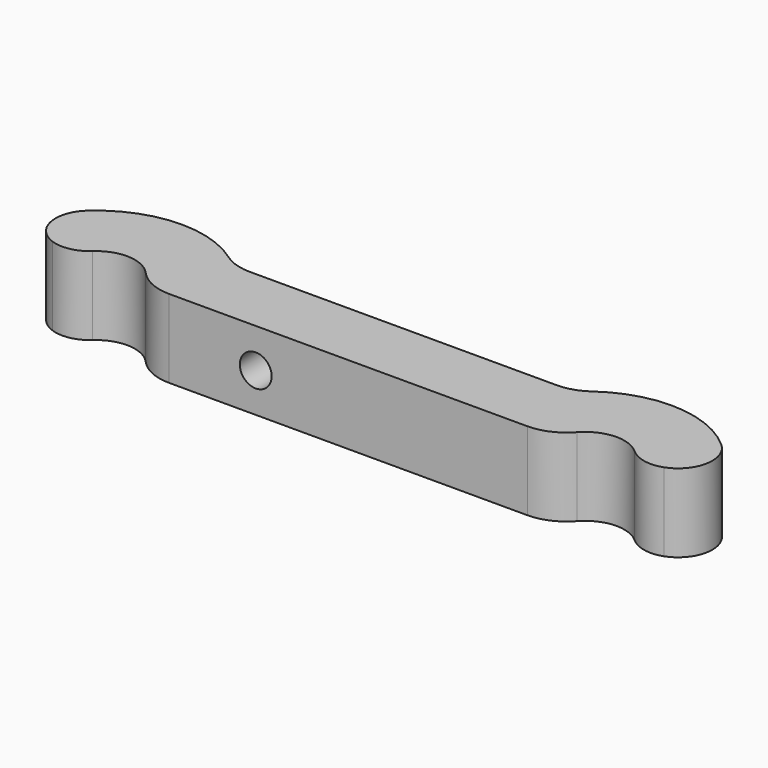
from build123d import *

# Parameters (mm, degrees)
F2_DEPTH = 8
F4_R     = 5
F5_R     = 3.49999
F3_R     = 1.625
F8_DEPTH = 7.001


# Not quite as in the source:
# - a fillet or chamfer is up to 0.001 mm smaller than in the source, because OpenCascade refuses the exact size


with BuildPart() as f2:
    # F1 (on Top) → F2 (new body)
    with BuildSketch(Plane.XY):
        with BuildLine():
            Line((0, 7), (-17.4501655647, 7))
            ThreePointArc((-17.4501655647, 7), (-27.535987639, 9.7036800538), (-35.3366188286, 2.7622215766))
            Line((-35.3366188286, 2.7622215766), (-28.7587704831, 0.3680805733))
            ThreePointArc((-28.7587704831, 0.3680805733), (-24.8073034208, 2.9953558075), (-21.1270166538, 0))
            Line((-21.1270166538, 0), (0, 0))
            Line((0, 0), (0, 7))
        make_face()
    extrude(amount=F2_DEPTH)

    # F4
    f4_edges = [f2.edges().sort_by_distance(p)[0] for p in [
        (-17.450166, 7, 4),
        (-21.127017, 0, 4),
    ]]
    fillet(f4_edges, radius=F4_R)

    # F5 (radius 3.5 in the source; OpenCascade refuses exactly that, so slightly less here)
    f5_edges = [f2.edges().sort_by_distance(p)[0] for p in [
        (-35.336619, 2.762222, 4),
        (-28.75877, 0.368081, 4),
    ]]
    fillet(f5_edges, radius=F5_R)

    # F7: F2 across face


with BuildPart() as f2_1:
    add(f2.part)
    add(f2.part.mirror(Plane(origin=(0, 3.5, 4), x_dir=(0, 1, 0), z_dir=(1, 0, 0))))

    # F3 (on face) → F8 (cut, through all)
    with BuildSketch(Plane(origin=(0, 7, 0), x_dir=(-1, 0, 0), z_dir=(0, 1, 0))):
        with Locations((9.4501655647, 4)):
            Circle(F3_R)
    extrude(amount=-F8_DEPTH, mode=Mode.SUBTRACT)


solid = f2_1.part
